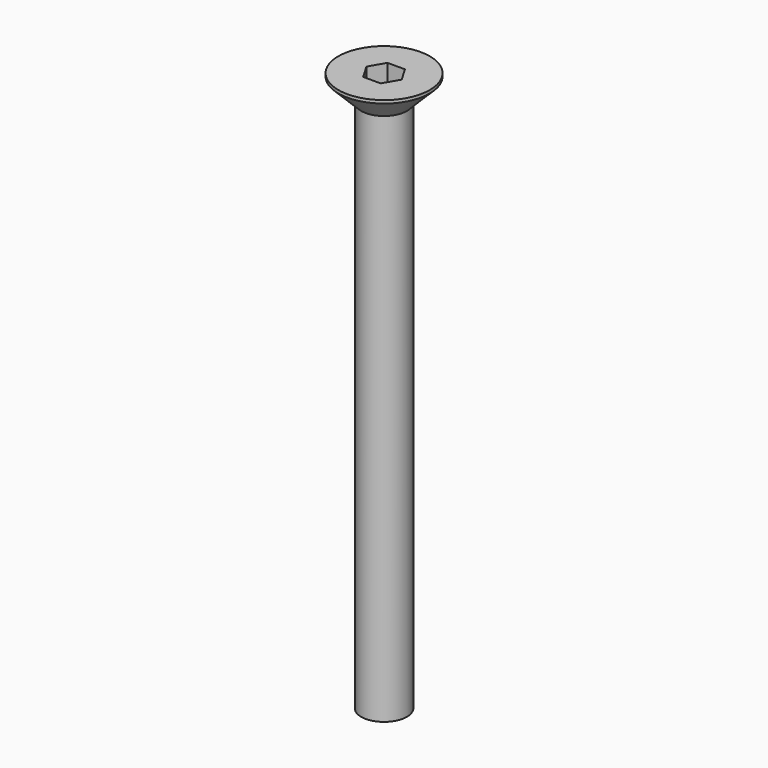
from build123d import *

# Parameters (mm, degrees)
F0_R     = 1.5
F1_DEPTH = 35
F0_R_2   = 3
F2_DEPTH = 1.7
F4_DEPTH = 1.5
F5_SIZE  = 1.49999


# Not quite as in the source:
# - a fillet or chamfer is up to 0.001 mm smaller than in the source, because OpenCascade refuses the exact size


with BuildPart() as f1:
    # F0 (on Top) → F1 (new body)
    with BuildSketch(Plane.XY):
        Circle(F0_R)
    extrude(amount=-F1_DEPTH)

    # F0 (on Top) → F2 (join)
    with BuildSketch(Plane.XY):
        Circle(F0_R_2)
        Circle(F0_R, mode=Mode.SUBTRACT)
        Circle(F0_R)
    extrude(amount=F2_DEPTH)

    # F3 (on face) → F4 (cut)
    with BuildSketch(Plane.XY.offset(1.7)):
        Polygon((-0.5773502692, -1), (0.5773502692, -1), (1.1547005384, 0), (0.5773502692, 1), (-0.5773502692, 1), (-1.1547005384, 0), align=None)
    extrude(amount=-F4_DEPTH, mode=Mode.SUBTRACT)

    # F5 (size 1.5 in the source; OpenCascade refuses exactly that, so slightly less here)
    f5_edges = [f1.edges().sort_by_distance(p)[0] for p in [
        (-3, 0, 0),
    ]]
    chamfer(f5_edges, length=F5_SIZE)


solid = f1.part
